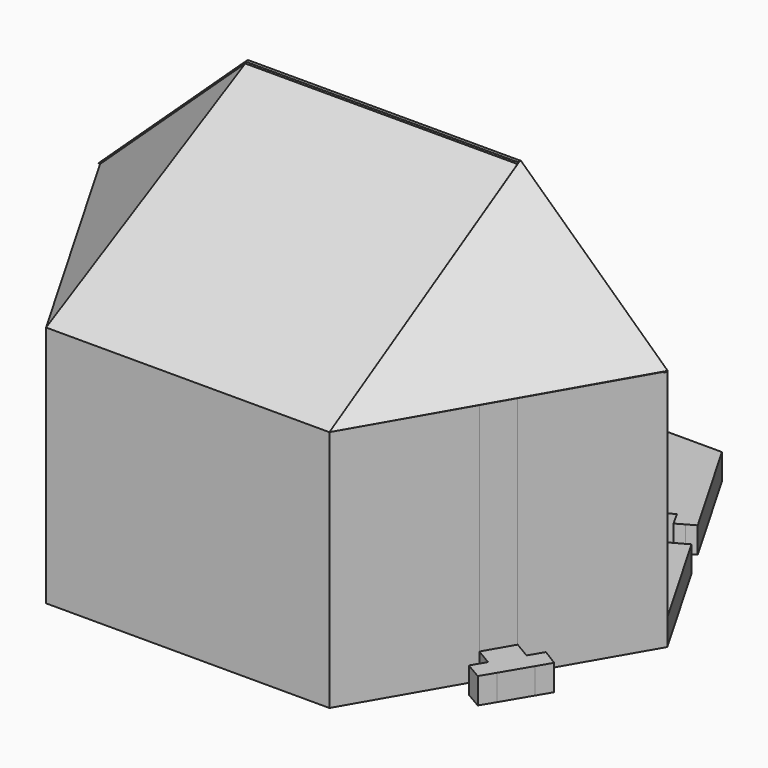
from build123d import *

# Parameters (mm, degrees)
F0_W      = 50
F0_H      = 12.5
F1_DEPTH  = 8
F2_DEPTH  = 75
F4_DEPTH  = 8
F7_DEPTH  = 3
F8_DEPTH  = 1
F11_DEPTH = 3
F14_DEPTH = 3
F15_DEPTH = 8
F16_DEPTH = 8
F17_DEPTH = 8


# Not quite as in the source:
# - a feature names something its author has since deleted; it is built from what else it names


with BuildPart() as f1:
    # F0 (on Top) → F1 (new body)
    with BuildSketch(Plane.XY):
        Polygon((57.9695070384, 39.3207329262), (60.5095952989, 40.7487522591), (42.0179491924, 72.7772228311), (-42.0179491924, 72.7772228311), (-84.0358983849, 0), (-42.0179491924, -72.7772228311), (42.0179491924, -72.7772228311), (84.0358983849, 0), (65.5269237886, 32.0584843966), (65.5097997054, 32.0881441788), (62.870004896, 30.6039762231), (65.3204122546, 26.2455930623), (60.0654171506, 23.2910848888), (57.615009792, 27.6494680496), (55.164720758, 32.0079177338), (52.7144317239, 36.366367418), (50.2642610162, 40.7248836223), (55.5194165334, 43.6791064608), align=None)
        with Locations((0, 54.5829171234)):
            Rectangle(F0_W, F0_H, mode=Mode.SUBTRACT)
    extrude(amount=F1_DEPTH)

    # F0 (on Top) → F2 (join)
    with BuildSketch(Plane.XY):
        Polygon((-84.0358983849, 0), (-87.5, 0), (-43.75, -75.7772228311), (43.75, -75.7772228311), (63.1745123486, -42.1329805311), (68.1246734519, -33.5590499945), (87.5, 0), (84.0358983849, 0), (42.0179491924, -72.7772228311), (-42.0179491924, -72.7772228311), align=None)
    extrude(amount=F2_DEPTH)

    # F0 (on Top) → F4 (join)
    with BuildSketch(Plane.XY):
        Polygon((43.75, 75.7772228311), (-43.75, 75.7772228311), (-65.625, 37.8886114156), (-68.125, 33.5584843966), (-87.5, 0), (-84.0358983849, 0), (-42.0179491924, 72.7772228311), (42.0179491924, 72.7772228311), (60.5095952989, 40.7487522591), (63.1248363216, 42.2190219338), align=None)
    extrude(amount=F4_DEPTH)

    # F6 (on face) → F7 (join)
    with BuildSketch(Plane(origin=(0, -50.1312366318, 89.3836679776), x_dir=(1, 0, 0), z_dir=(0, 0.4891706574, -0.872188092))):
        Polygon((43.75, 29.4041920927), (0, 29.4041920927), (-43.75, 29.4041920927), (-42.01795, -57.4775522498), (42.01795, -57.4775522498), align=None)
    extrude(amount=F7_DEPTH)

    # F3 (on Front) → F8 (join)
    with BuildSketch(Plane.XZ):
        Polygon((-42.01795, 114.5), (0, 114.5), (42.01795, 114.5), (84.0359, 75), (87.5, 75), (42.01795, 117.5), (0, 117.5), (-42.01795, 117.5), (-87.5, 75), (-84.0359, 75), align=None)
    extrude(amount=F8_DEPTH)

    # F10 (on face) → F11 (join)
    with BuildSketch(Plane(origin=(-67.6846727043, -39.0777640058, 72.4338274863), x_dir=(0.7723629594, -0.3015876344, 0.5590173143), z_dir=(-0.6351814378, -0.3667221741, 0.6797495039))):
        Polygon((33.2314262259, 55.789645187), (-25.6554603702, 35.6104118215), (30.9888924807, -31.0804218073), align=None)
    extrude(amount=-F11_DEPTH)

    # F13 (on face) → F14 (join)
    with BuildSketch(Plane(origin=(67.6756688636, -39.5950852503, 72.4241918832), x_dir=(0.7733047167, 0.3041472681, -0.556322078), z_dir=(-0.6340345536, 0.3709553614, -0.6785221475))):
        Polygon((-30.939509805, 30.5117392321), (-32.8751652468, -56.3649154418), (25.9400068576, -35.9776056011), align=None)
    extrude(amount=F14_DEPTH)

    # F0 (on Top) → F15 (join)
    with BuildSketch(Plane.XY):
        with Locations((0, 54.5829171234)):
            Rectangle(F0_W, F0_H)
    extrude(amount=F15_DEPTH)

    # F0 (on Top) → F16 (join)
    with BuildSketch(Plane.XY):
        Polygon((75.878553621, -32.3439069124), (73.3299584755, -36.6440801541), (78.4478092981, -39.6772904524), (80.9460908184, -35.4620099819), align=None)
        Polygon((73.3299584755, -36.6440801541), (68.1246734519, -33.5590499945), (63.1745123486, -42.1329805311), (68.2616414678, -45.1481695385), (73.3985163623, -48.1928433322), (78.4478092981, -39.6772904524), align=None)
        Polygon((73.3985163623, -48.1928433322), (68.2616414678, -45.1481695385), (65.7363801019, -49.4055813149), (70.880193178, -52.396181094), align=None)
    extrude(amount=F16_DEPTH)

    # F0 (on Top) → F17 (join)
    with BuildSketch(Plane.XY):
        Polygon((87.5, 0), (68.125, 33.5584843966), (65.5269237886, 32.0584843966), (84.0358983849, 0), align=None)
    extrude(amount=F17_DEPTH)


solid = f1.part
